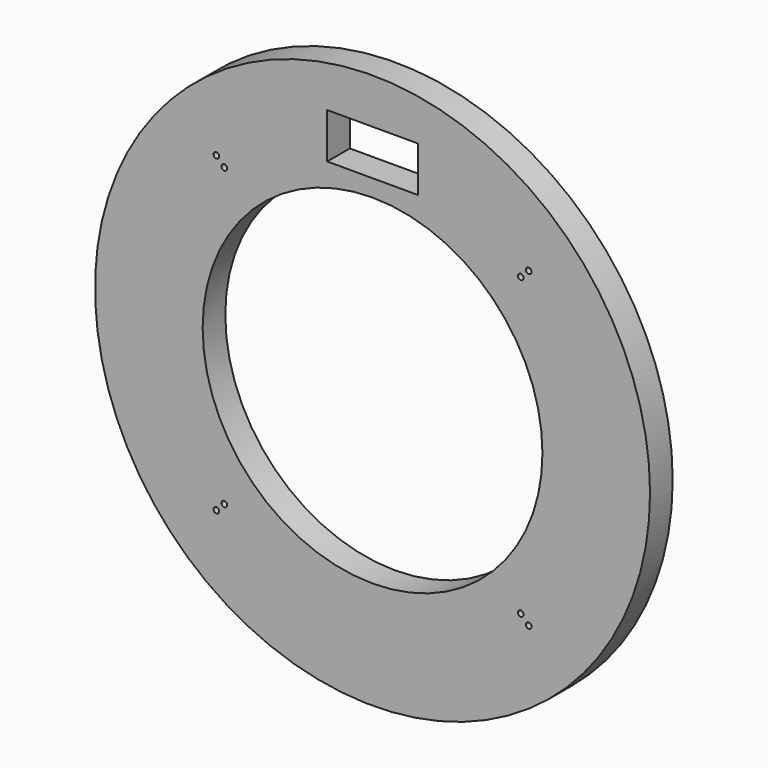
from build123d import *

# Parameters (mm, degrees)
F0_R     = 245
F0_R_2   = 2.5
F0_R_3   = 150
F0_W     = 25
F0_H     = 10
F1_DEPTH = 25


with BuildPart() as f1:
    # F0 (on Front) → F1 (new body)
    with BuildSketch(Plane.XZ):
        Circle(F0_R)
        with Locations((-137.8858223314, -137.8858223314)):
            Circle(F0_R_2, mode=Mode.SUBTRACT)
        with Locations((-130.8147545195, -130.8147545195)):
            Circle(F0_R_2, mode=Mode.SUBTRACT)
        with Locations((137.8858223314, -137.8858223314)):
            Circle(F0_R_2, mode=Mode.SUBTRACT)
        with Locations((130.8147545195, -130.8147545195)):
            Circle(F0_R_2, mode=Mode.SUBTRACT)
        with Locations((-130.8147545195, 130.8147545195)):
            Circle(F0_R_2, mode=Mode.SUBTRACT)
        with Locations((-137.8858223314, 137.8858223314)):
            Circle(F0_R_2, mode=Mode.SUBTRACT)
        Circle(F0_R_3, mode=Mode.SUBTRACT)
        Polygon((40, 205), (40, 165), (-40, 165), (-40, 205), (-12.5, 205), (-12.5, 215), (12.5, 215), (12.5, 205), align=None, mode=Mode.SUBTRACT)
        with Locations((130.8147545195, 130.8147545195)):
            Circle(F0_R_2, mode=Mode.SUBTRACT)
        with Locations((137.8858223314, 137.8858223314)):
            Circle(F0_R_2, mode=Mode.SUBTRACT)
        with Locations((0, 210)):
            Rectangle(F0_W, F0_H)
    extrude(amount=F1_DEPTH)


solid = f1.part
